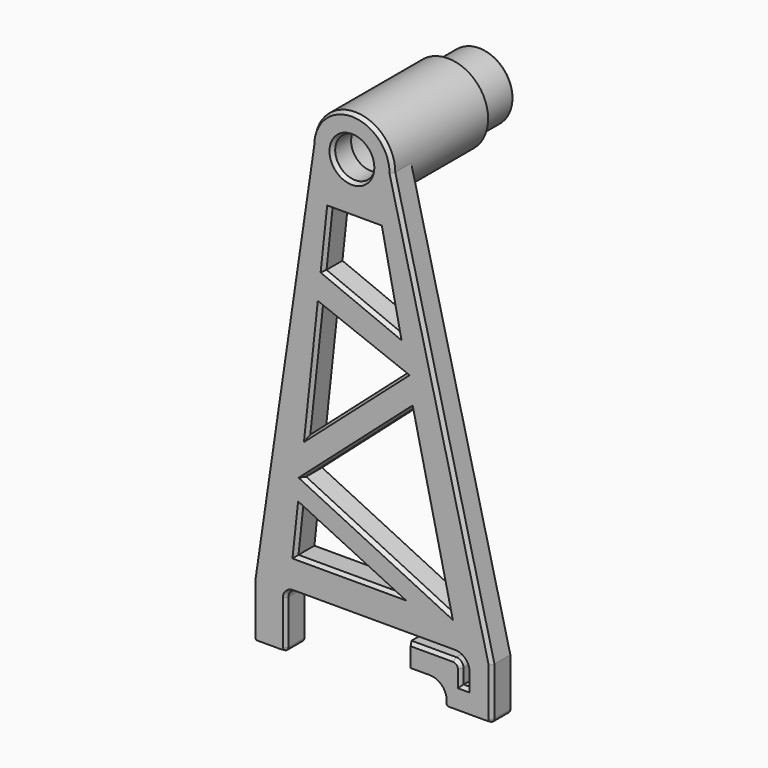
from build123d import *
from build123d import SkipClean  # not in build123d's __all__

# Parameters (mm, degrees)
F1_DEPTH = 7.62
F2_R     = 12.7
F2_R_2   = 9.398
F3_DEPTH = 38.1
F4_R     = 10.668
F4_R_2   = 9.398
F5_DEPTH = 12.7
F6_R     = 6.35
F7_DEPTH = 25.4
F8_SIZE2 = 1.3198227154
F8_SIZE  = 0.762
F9_R     = 0.762


# Not quite as in the source:
# - after a boolean that leaves OpenCascade's solid faulty, fix() repairs it


with BuildPart() as f1:
    # F0 (on Front) → F1 (new body)
    with BuildSketch(Plane.XZ):
        with BuildLine():
            ThreePointArc((-21.1420084076, -2.54), (-20.3980596318, -0.7439487758), (-18.6020084076, 0))
            Line((-18.6020084076, 0), (32.7059915924, 0))
            ThreePointArc((32.7059915924, 0), (35.4000684287, -1.1159231637), (36.5159915924, -3.81))
            Line((36.5159915924, -3.81), (36.5159915924, -8.89))
            Line((36.5159915924, -8.89), (34.3569915924, -8.89))
            Line((34.3569915924, -8.89), (34.3569915924, -4.318))
            ThreePointArc((34.3569915924, -4.318), (33.6874376942, -2.7015538982), (32.0709915924, -2.032))
            Line((32.0709915924, -2.032), (29.2769915924, -2.032))
            Line((29.2769915924, -2.032), (17.8469915924, -2.032))
            Line((17.8469915924, -2.032), (17.8469915924, -9.652))
            Line((17.8469915924, -9.652), (24.7049915924, -9.652))
            ThreePointArc((24.7049915924, -9.652), (27.937883796, -10.9911077964), (29.2769915924, -14.224))
            Line((29.2769915924, -14.224), (29.2769915924, -15.24))
            ThreePointArc((29.2769915924, -15.24), (29.6489659803, -16.1380256121), (30.5469915924, -16.51))
            Line((30.5469915924, -16.51), (42.8659915924, -16.51))
            ThreePointArc((42.8659915924, -16.51), (43.7640172045, -16.1380256121), (44.1359915924, -15.24))
            Line((44.1359915924, -15.24), (44.1359915924, 0))
            Line((44.1359915924, 0), (12.7, 127))
            ThreePointArc((12.7, 127), (0, 139.7), (-12.7, 127))
            Line((-12.7, 127), (-31.3020084076, 0))
            Line((-31.3020084076, 0), (-31.3020084076, -16.51))
            ThreePointArc((-31.3020084076, -16.51), (-30.9300340197, -17.4080256121), (-30.0320084076, -17.78))
            Line((-30.0320084076, -17.78), (-22.4120084076, -17.78))
            ThreePointArc((-22.4120084076, -17.78), (-21.5139827955, -17.4080256121), (-21.1420084076, -16.51))
            Line((-21.1420084076, -16.51), (-21.1420084076, -2.54))
        make_face()
        Polygon((13.8583155349, 10.2559253573), (-17.4904800951, 10.2559253573), (-17.9861974368, 10.2559253573), (-16.4103638381, 24.8740110546), align=None, mode=Mode.SUBTRACT)
        Polygon((30.8991490559, 10.2559253573), (-15.5502194539, 32.8530669212), (18.8005114427, 63.1991239488), align=None, mode=Mode.SUBTRACT)
        Polygon((16.8689347681, 72.4665825348), (-14.2382610105, 45.0233372929), (-10.1512422372, 82.9362176403), align=None, mode=Mode.SUBTRACT)
        Polygon((-7.1419274588, 110.8518689871), (8.8684540242, 110.8518689871), (14.6986516415, 82.8793242388), (-9.1010310551, 92.6784119132), align=None, mode=Mode.SUBTRACT)
    extrude(amount=F1_DEPTH)

    # F2 (on face) → F3 (join)
    with BuildSketch(Plane.XZ.offset(7.62)):
        with Locations((0, 127)):
            Circle(F2_R)
        with Locations((0, 127)):
            Circle(F2_R_2, mode=Mode.SUBTRACT)
    extrude(amount=-F3_DEPTH)

    # F4 (on face) → F5 (join)
    with BuildSketch(Plane(origin=(0, 30.48, 0), x_dir=(-1, 0, 0), z_dir=(0, 1, 0))):
        with Locations((0, 127)):
            Circle(F4_R)
        with Locations((0, 127)):
            Circle(F4_R_2, mode=Mode.SUBTRACT)
    with SkipClean():  # cleaning this boolean's faces spoils the solid; the shape is the same uncleaned
        extrude(amount=F5_DEPTH)

    # F6 (on face) → F7 (cut)
    with BuildSketch(Plane.XZ.offset(7.62)):
        with Locations((0, 127)):
            Circle(F6_R)
    extrude(amount=-F7_DEPTH, mode=Mode.SUBTRACT)

    add(f1.part.fix(), mode=Mode.REPLACE)

    # F8
    f8_edges = [f1.edges().sort_by_distance(p)[0] for p in [
        (-22.001004, -7.62, 63.5),
        (-31.302008, -7.62, -8.255),
        (-30.930034, -7.62, -17.408026),
        (-26.222008, -7.62, -17.78),
        (-21.513983, -7.62, -17.408026),
        (-21.142008, -7.62, -9.525),
        (-20.39806, -7.62, -0.743949),
        (7.051992, -7.62, 0),
        (35.400068, -7.62, -1.115923),
        (36.515992, -7.62, -6.35),
        (35.436492, -7.62, -8.89),
        (34.356992, -7.62, -6.604),
        (33.687438, -7.62, -2.701554),
        (24.958992, -7.62, -2.032),
        (17.846992, -7.62, -5.842),
        (21.275992, -7.62, -9.652),
        (27.937884, -7.62, -10.991108),
        (29.276992, -7.62, -14.732),
        (29.648966, -7.62, -16.138026),
        (36.706492, -7.62, -16.51),
        (43.764017, -7.62, -16.138026),
        (44.135992, -7.62, -7.62),
        (28.417996, -7.62, 63.5),
        (0, -7.62, 139.7),
        (-17.198281, -7.62, 17.564968),
        (-1.276024, -7.62, 17.564968),
        (-2.063941, -7.62, 10.255925),
        (1.315337, -7.62, 58.74496),
        (-12.194752, -7.62, 63.979777),
        (3.358846, -7.62, 77.7014),
        (24.84983, -7.62, 36.727525),
        (7.674465, -7.62, 21.554496),
        (1.625146, -7.62, 48.026095),
        (0.863263, -7.62, 110.851869),
        (11.783553, -7.62, 96.865597),
        (2.79881, -7.62, 87.778868),
        (-8.121479, -7.62, 101.76514),
        (-6.35, -7.62, 127),
    ]]
    f8_side = f1.faces().sort_by_distance((-20.273277, -7.62, 63.246935))[0]
    chamfer(f8_edges, length=F8_SIZE, length2=F8_SIZE2, reference=f8_side)

    # F9
    f9_edges = [f1.edges().sort_by_distance(p)[0] for p in [
        (10.668, 43.18, 127),
    ]]
    fillet(f9_edges, radius=F9_R)


solid = f1.part
